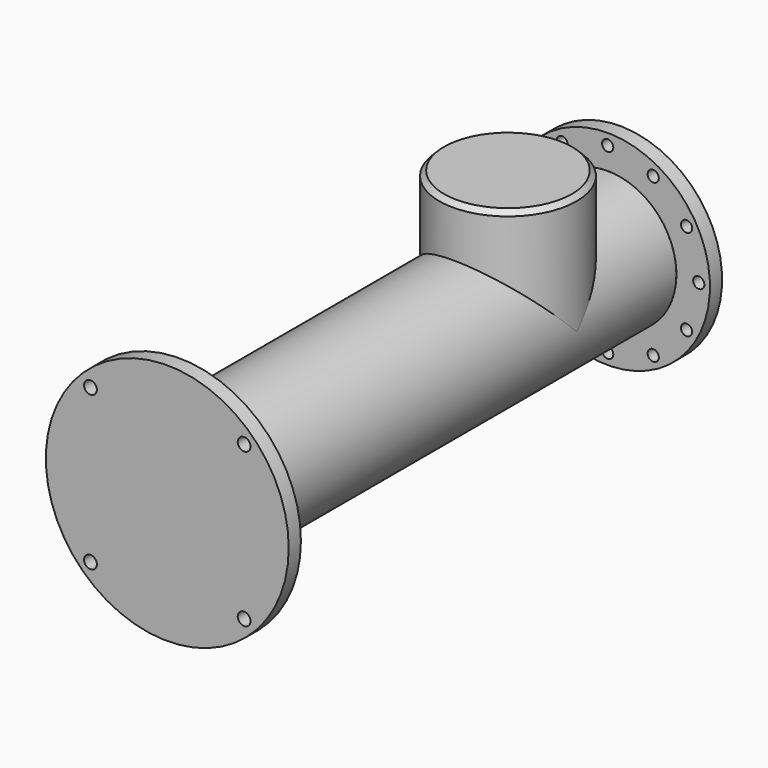
from build123d import *

# Parameters (mm, degrees)
F0_R      = 136.525
F1_DEPTH  = 1063.5615
F2_R      = 132.334
F3_DEPTH  = 1051.19424
F4_R      = 241.3
F4_R_2    = 12.7
F5_DEPTH  = 30.226
F6_R      = 203.2
F6_R_2    = 11.1125
F6_R_3    = 136.525
F7_DEPTH  = 30.226
F8_R      = 136.525
F8_R_2    = 127
F9_DEPTH  = 238.125
F10_SIZE  = 9.52499
F11_R     = 127
F12_DEPTH = 25.4


# Not quite as in the source:
# - a fillet or chamfer is up to 0.001 mm smaller than in the source, because OpenCascade refuses the exact size


with BuildPart() as f1:
    # F0 (on Front) → F1 (new body)
    with BuildSketch(Plane.XZ):
        Circle(F0_R)
    extrude(amount=F1_DEPTH)

    # F2 (on face) → F3 (cut)
    with BuildSketch(Plane.XZ.offset(1063.5615)):
        Circle(F2_R)
    extrude(amount=-F3_DEPTH, mode=Mode.SUBTRACT)

    # F4 (on face) → F5 (join)
    with BuildSketch(Plane.XZ.offset(1063.5615)):
        Circle(F4_R)
        with Locations((-152.6643540582, -152.6643540582)):
            Circle(F4_R_2, mode=Mode.SUBTRACT)
        with Locations((152.6643540582, -152.6643540582)):
            Circle(F4_R_2, mode=Mode.SUBTRACT)
        with Locations((-152.6643540582, 152.6643540582)):
            Circle(F4_R_2, mode=Mode.SUBTRACT)
        with Locations((152.6643540582, 152.6643540582)):
            Circle(F4_R_2, mode=Mode.SUBTRACT)
    extrude(amount=F5_DEPTH)

    # F8 (on Top) → F9 (join)
    with BuildSketch(Plane.XY):
        with Locations((0, -247.65)):
            Circle(F8_R)
        with Locations((0, -247.65)):
            Circle(F8_R_2, mode=Mode.SUBTRACT)
    extrude(amount=F9_DEPTH)

    # F10 (size 9.525 in the source; OpenCascade refuses exactly that, so slightly less here)
    f10_edges = [f1.edges().sort_by_distance(p)[0] for p in [
        (-136.525, -247.65, 238.125),
    ]]
    chamfer(f10_edges, length=F10_SIZE)

    # F11 (on Top) → F12 (cut)
    with BuildSketch(Plane.XY):
        with Locations((0, -247.65)):
            Circle(F11_R)
    extrude(amount=-F12_DEPTH, mode=Mode.SUBTRACT)


with BuildPart() as f7:
    # F6 (on face) → F7 (new body)
    with BuildSketch(Plane(origin=(0, 0, 0), x_dir=(-1, 0, 0), z_dir=(0, 1, 0))):
        Circle(F6_R)
        with Locations((-90.4875, -156.7289474499)):
            Circle(F6_R_2, mode=Mode.SUBTRACT)
        with Locations((0, -180.975)):
            Circle(F6_R_2, mode=Mode.SUBTRACT)
        with Locations((-156.7289474499, -90.4875)):
            Circle(F6_R_2, mode=Mode.SUBTRACT)
        with Locations((-180.975, 0)):
            Circle(F6_R_2, mode=Mode.SUBTRACT)
        Circle(F6_R_3, mode=Mode.SUBTRACT)
        with Locations((90.4875, -156.7289474499)):
            Circle(F6_R_2, mode=Mode.SUBTRACT)
        with Locations((156.7289474499, -90.4875)):
            Circle(F6_R_2, mode=Mode.SUBTRACT)
        with Locations((180.975, 0)):
            Circle(F6_R_2, mode=Mode.SUBTRACT)
        with Locations((-156.7289474499, 90.4875)):
            Circle(F6_R_2, mode=Mode.SUBTRACT)
        with Locations((-90.4875, 156.7289474499)):
            Circle(F6_R_2, mode=Mode.SUBTRACT)
        with Locations((0, 180.975)):
            Circle(F6_R_2, mode=Mode.SUBTRACT)
        with Locations((156.7289474499, 90.4875)):
            Circle(F6_R_2, mode=Mode.SUBTRACT)
        with Locations((90.4875, 156.7289474499)):
            Circle(F6_R_2, mode=Mode.SUBTRACT)
    extrude(amount=F7_DEPTH)


solid = Compound([f1.part, f7.part])
